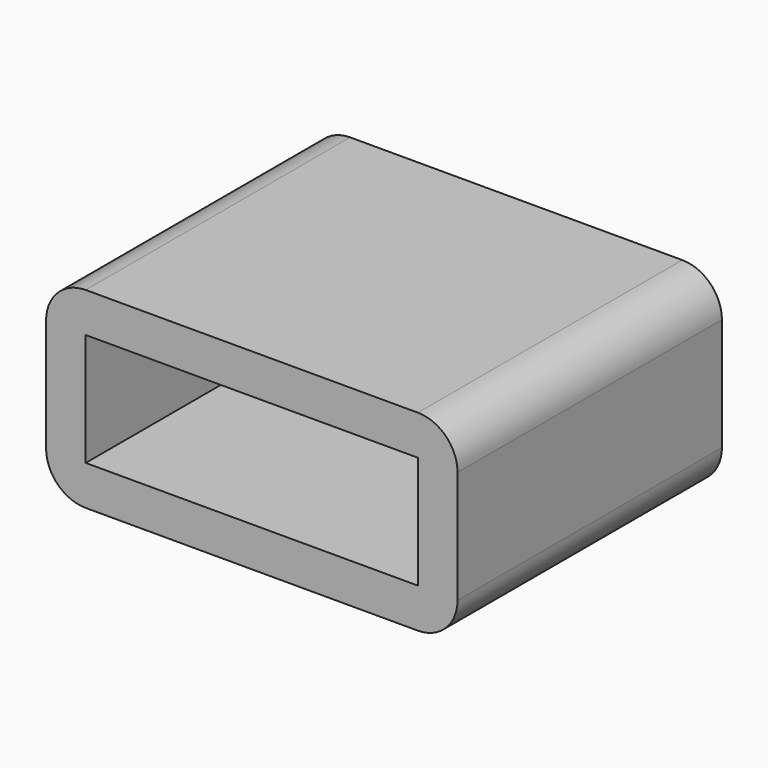
from build123d import *

# Parameters (mm, degrees)
F1_DEPTH = 25
F2_T     = 3


# Not quite as in the source:
# - a shell that OpenCascade refuses in one call is made with other operations: the cavity is built on its own and cut out


with BuildPart() as f1:
    # F0 (on Front) → F1 (new body)
    with BuildSketch(Plane.XZ):
        with BuildLine():
            Line((-30.3064525574, 35.3830642998), (-55.4274195135, 35.3830642998))
            ThreePointArc((-55.4274195135, 35.3830642998), (-57.548739857, 34.5043846434), (-58.4274195135, 32.3830642998))
            Line((-58.4274195135, 32.3830642998), (-58.4274195135, 23.8669360727))
            ThreePointArc((-58.4274195135, 23.8669360727), (-57.548739857, 21.7456157291), (-55.4274195135, 20.8669360727))
            Line((-55.4274195135, 20.8669360727), (-30.3064525574, 20.8669360727))
            ThreePointArc((-30.3064525574, 20.8669360727), (-28.1851322139, 21.7456157291), (-27.3064525574, 23.8669360727))
            Line((-27.3064525574, 23.8669360727), (-27.3064525574, 32.3830642998))
            ThreePointArc((-27.3064525574, 32.3830642998), (-28.1851322139, 34.5043846434), (-30.3064525574, 35.3830642998))
        make_face()
    extrude(amount=F1_DEPTH)

    # F2: shell of thickness 3, made by hand


with BuildPart() as f2_core1:
    # F2_t2: copy of F1
    add(f1.part)

    # the walls: a layer under each face that stays
    f2_faces = [f2_core1.faces().sort_by_distance(p)[0] for p in [
        (-42.8669360355, -12.5, 35.3830642998),
        (-58.4274195135, -12.5, 28.1250001863),
        (-42.8669360355, -12.5, 20.8669360727),
        (-27.3064525574, -12.5, 28.1250001863),
        (-42.8669360355, 0, 28.1250001863),
    ]]
    thicken(f2_faces, amount=-F2_T, mode=Mode.SUBTRACT)


with BuildPart() as f1_1:
    add(f1.part)

    # what is left inside the walls is the cavity
    f2_cavity = [f2_core1.part.solids().sort_by_distance(p)[0] for p in [
        (-42.866936, -17.666667, 23.896936),
    ]]
    add(f2_cavity, mode=Mode.SUBTRACT)


solid = f1_1.part
